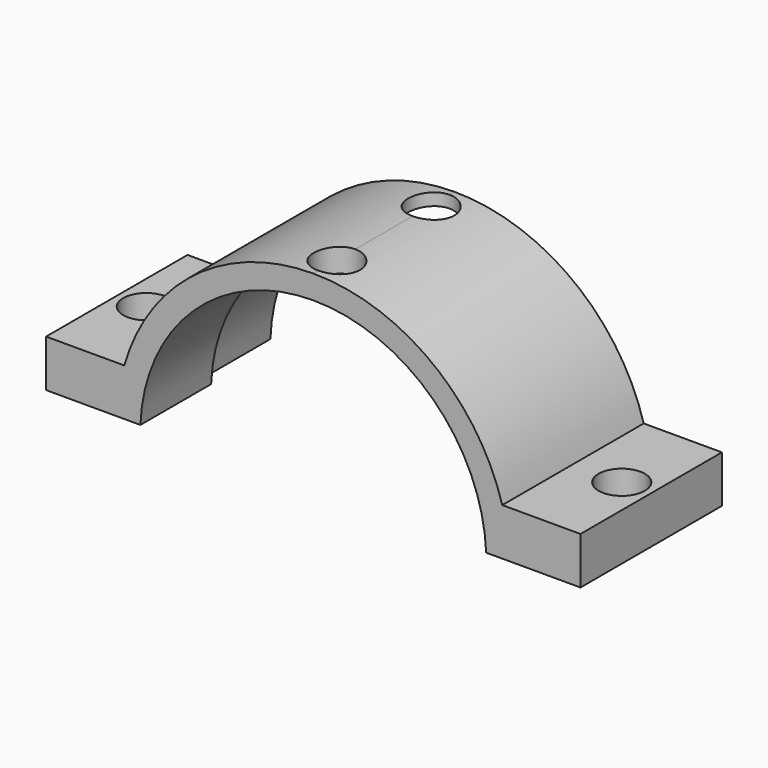
from build123d import *

# Parameters (mm, degrees)
F1_DEPTH = 19.05
F3_DEPTH = 9.525
F5_R     = 2.4892
F6_DEPTH = 25.4


# Not quite as in the source:
# - a length typed as a fraction of an inch, garbled in the dataset ("3 / 203.2 mm" for 3/8 in), is restored


with BuildPart() as f1:
    # F0 (on Front) → F1 (new body)
    with BuildSketch(Plane.XZ):
        with BuildLine():
            ThreePointArc((0, 18.6436), (12.9107977631, 13.4497257251), (18.6280212841, 0.762))
            Line((18.6280212841, 0.762), (28.7880212841, 0.762))
            Line((28.7880212841, 0.762), (28.7880212841, 5.842))
            Line((28.7880212841, 5.842), (20.3621203454, 5.842))
            ThreePointArc((20.3621203454, 5.842), (12.7473588982, 16.9189169299), (0, 21.1836))
            Line((0, 21.1836), (0, 18.6436))
        make_face()
    extrude(amount=F1_DEPTH)

    # F2 (on face) → F3 (cut)
    with BuildSketch(Plane(origin=(0, 0, 0), x_dir=(-1, 0, 0), z_dir=(0, 1, 0))):
        with BuildLine():
            ThreePointArc((0, 19.8755), (-14.0541008295, 14.0541008295), (-19.8755, 0))
            Line((-19.8755, 0), (0, 0))
            Line((0, 0), (0, 19.8755))
        make_face()
    extrude(amount=-F3_DEPTH, mode=Mode.SUBTRACT)

    # F4: F1 across face


with BuildPart() as f1_1:
    add(f1.part)
    add(f1.part.mirror(Plane(origin=(0, -11.0496287129, 20.1229823432), x_dir=(0, -1, 0), z_dir=(-1, 0, 0))))

    # F5 (on Top) → F6 (cut)
    with BuildSketch(Plane.XY):
        with Locations((0, -15.875)):
            Circle(F5_R)
        with Locations((0, -3.175)):
            Circle(F5_R)
        with Locations((-25.6130212841, -9.525)):
            Circle(F5_R)
        with Locations((25.6130212841, -9.525)):
            Circle(F5_R)
    extrude(amount=F6_DEPTH, mode=Mode.SUBTRACT)


solid = f1_1.part
